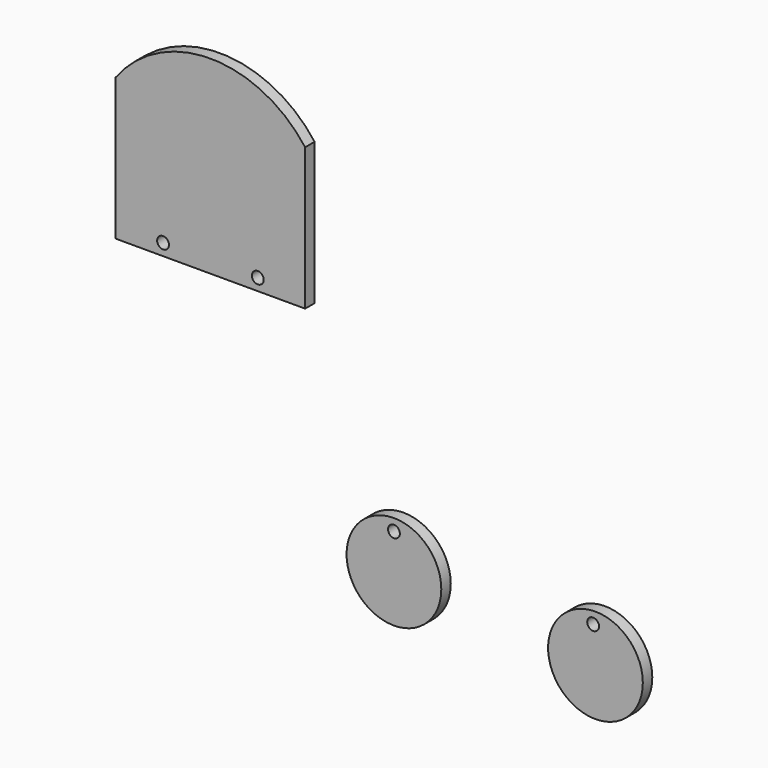
from build123d import *

# Parameters (mm, degrees)
F0_R     = 3.175
F1_DEPTH = 6.35
F0_R_2   = 25.4


# Not quite as in the source:
# - a feature names something its author has since deleted; it is built from what else it names


with BuildPart() as f1:
    # F0 (on Front) → F1 (new body)
    with BuildSketch(Plane.XZ):
        with BuildLine():
            Line((-183.6576171661, 195.2901095029), (-183.6576171661, 119.0901095029))
            Line((-183.6576171661, 119.0901095029), (-82.0576171661, 119.0901095029))
            Line((-82.0576171661, 119.0901095029), (-82.0576171661, 195.2901095029))
            ThreePointArc((-82.0576171661, 195.2901095029), (-132.8576171661, 220.6901095029), (-183.6576171661, 195.2901095029))
        make_face()
        with Locations((-158.2576171661, 125.4401095029)):
            Circle(F0_R, mode=Mode.SUBTRACT)
        with Locations((-107.4576171661, 125.4401095029)):
            Circle(F0_R, mode=Mode.SUBTRACT)
    extrude(amount=F1_DEPTH)


with BuildPart() as f1b:
    # F0 (on Front) → F1, piece 2 (new body)
    with BuildSketch(Plane.XZ):
        with Locations((-34.4394389217, 10.3405317959)):
            Circle(F0_R_2)
        with Locations((-34.4394389217, 29.3905317959)):
            Circle(F0_R, mode=Mode.SUBTRACT)
    extrude(amount=F1_DEPTH)


with BuildPart() as f1c:
    # F0 (on Front) → F1, piece 3 (new body)
    with BuildSketch(Plane.XZ):
        with Locations((73.6421495676, 1.3085657265)):
            Circle(F0_R_2)
        with Locations((72.3918600443, 20.3174919484)):
            Circle(F0_R, mode=Mode.SUBTRACT)
    extrude(amount=F1_DEPTH)


solid = Compound([f1.part, f1b.part, f1c.part])
